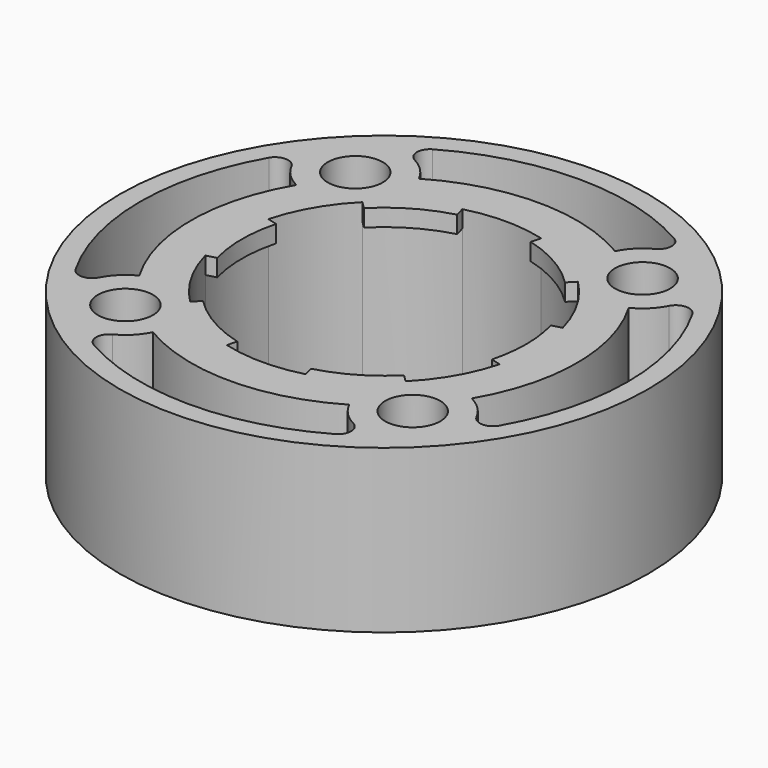
from build123d import *

# Parameters (mm, degrees)
F0_R            = 20.6375
F0_R_2          = 2.15265
F1_DEPTH        = 12.7
F3_DEPTH        = 12.7
F4_COUNT        = 6
F4_ANGLE        = 300
F6_R            = 11.90625
F7_DEPTH        = 11.36015
F9_DEPTH        = 12.7
F9_COPIES_COUNT = 4
F10_R           = 1.0241935484


# Not quite as in the source:
# - a pattern or mirror of a feature is missing from the dataset's text; its kind, count and spacing are read off the source's solid


with BuildPart() as f1:
    # F0 (on Top) → F1 (new body)
    with BuildSketch(Plane.XY):
        Circle(F0_R)
        with Locations((-11.2253201513, -11.2253201513)):
            Circle(F0_R_2, mode=Mode.SUBTRACT)
        with Locations((11.2253201513, -11.2253201513)):
            Circle(F0_R_2, mode=Mode.SUBTRACT)
        with Locations((-11.2253201513, 11.2253201513)):
            Circle(F0_R_2, mode=Mode.SUBTRACT)
        with BuildLine():
            ThreePointArc((0, 11.1125), (7.8577241059, 7.8577241059), (11.1125, 0))
            ThreePointArc((11.1125, 0), (-7.8577241059, -7.8577241059), (0, 11.1125))
        make_face(mode=Mode.SUBTRACT)
        with Locations((11.2253201513, 11.2253201513)):
            Circle(F0_R_2, mode=Mode.SUBTRACT)
    extrude(amount=F1_DEPTH)

    # F2 (on face) → F3 (cut, through all)
    with BuildSketch(Plane.XY.offset(12.7)):
        with BuildLine():
            ThreePointArc((-2.8761266387, 10.7338507446), (0, 11.1125), (2.8761266387, 10.7338507446))
            Line((2.8761266387, 10.7338507446), (3.0815642558, 11.5005543693))
            ThreePointArc((3.0815642558, 11.5005543693), (0, 11.90625), (-3.0815642558, 11.5005543693))
            Line((-3.0815642558, 11.5005543693), (-2.8761266387, 10.7338507446))
        make_face()
    f3 = extrude(amount=-F3_DEPTH, mode=Mode.SUBTRACT)

    # F4: F3 ×6 about axis
    f4_axis = Axis((0, 0, 0), (0, 0, -1))
    for i in range(1, F4_COUNT):
        add(f3.rotate(f4_axis, i * F4_ANGLE / (F4_COUNT - 1)), mode=Mode.SUBTRACT)

    # F6 (on face) → F7 (cut, through all)
    with BuildSketch(Plane(origin=(0, 0, 0), x_dir=(1, 0, 0), z_dir=(0, 0, -1))):
        Circle(F6_R)
    extrude(amount=-F7_DEPTH, mode=Mode.SUBTRACT)

    # F8 (on face) → F9 (cut, through all)
    with BuildSketch(Plane(origin=(0, 0, 0), x_dir=(1, 0, 0), z_dir=(0, 0, -1))):
        with BuildLine():
            ThreePointArc((11.5039191556, -15.1842795042), (9.251826165, -14.6686177057), (7.6685282311, -12.9860608474))
            ThreePointArc((7.6685282311, -12.9860608474), (0, -15.08125), (-7.6685282311, -12.9860608474))
            ThreePointArc((-7.6685282311, -12.9860608474), (-9.251826165, -14.6686177057), (-11.5039191556, -15.1842795042))
            ThreePointArc((-11.5039191556, -15.1842795042), (0, -19.05), (11.5039191556, -15.1842795042))
        make_face()
    f9 = extrude(amount=-F9_DEPTH, mode=Mode.SUBTRACT)

    # F9_copies: F9 ×4 about axis
    f9_copies_axis = Axis((0, 0, 0), (0, 0, 1))
    for i in range(1, F9_COPIES_COUNT):
        add(f9.rotate(f9_copies_axis, i * 360 / F9_COPIES_COUNT), mode=Mode.SUBTRACT)

    # F10
    f10_edges = [f1.edges().sort_by_distance(p)[0] for p in [
        (-11.503919, 15.18428, 6.35),
        (11.503919, 15.18428, 6.35),
        (11.503919, -15.18428, 6.35),
        (-11.503919, -15.18428, 6.35),
        (-15.18428, -11.503919, 6.35),
        (-15.18428, 11.503919, 6.35),
        (15.18428, 11.503919, 6.35),
        (15.18428, -11.503919, 6.35),
    ]]
    fillet(f10_edges, radius=F10_R)


solid = f1.part
